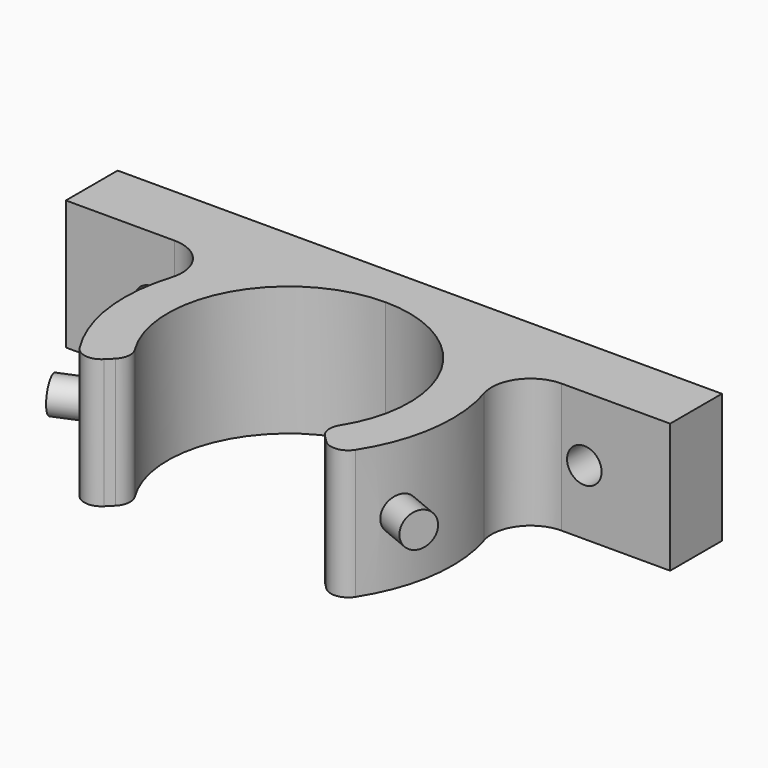
from build123d import *

# Parameters (mm, degrees)
F1_DEPTH  = 15
F2_R      = 2
F3_DEPTH  = 7.5
F4_ANGLE  = 90
F5_R      = 4.5
F6_R      = 2
F10_R     = 2
F11_DEPTH = 5


# Not quite as in the source:
# - a pattern or mirror of a feature is missing from the dataset's text; its kind, count and spacing are read off the source's solid


with BuildPart() as f1:
    # F0 (on Right) → F1 (new body)
    with BuildSketch(Plane.YZ):
        with BuildLine():
            ThreePointArc((-8.7152049129, 10.9565141959), (6.0822336037, 12.6097753505), (14, 0))
            ThreePointArc((14, 0), (6.0822336037, -12.6097753505), (-8.7152049129, -10.9565141959))
            Line((-8.7152049129, -10.9565141959), (-12.2675540951, -14.5088633781))
            ThreePointArc((-12.2675540951, -14.5088633781), (-0.4919673203, -18.993629673), (11.5, -15.1244834623))
            ThreePointArc((11.5, -15.1244834623), (17.0220445305, -8.4409715081), (19, 0))
            ThreePointArc((19, 0), (17.0220445305, 8.4409715081), (11.5, 15.1244834623))
            ThreePointArc((11.5, 15.1244834623), (-0.4919673203, 18.993629673), (-12.2675540951, 14.5088633781))
            Line((-12.2675540951, 14.5088633781), (-8.7152049129, 10.9565141959))
        make_face()
        with BuildLine():
            Line((11.5, 35), (11.5, 15.1244834623))
            ThreePointArc((11.5, 15.1244834623), (17.0220445305, 8.4409715081), (19, 0))
            Line((19, 0), (19, 35))
            Line((19, 35), (11.5, 35))
        make_face()
        with BuildLine():
            ThreePointArc((19, 0), (17.0220445305, -8.4409715081), (11.5, -15.1244834623))
            Line((11.5, -15.1244834623), (11.5, -35))
            Line((11.5, -35), (19, -35))
            Line((19, -35), (19, 0))
        make_face()
    extrude(amount=F1_DEPTH)

    # F2 (on face) → F3 (cut, through all)
    with BuildSketch(Plane.XZ.offset(-11.5)):
        with Locations((7.5, 25.0622417311)):
            Circle(F2_R)
        with Locations((7.5, -25.0622417311)):
            Circle(F2_R)
    extrude(amount=-F3_DEPTH, mode=Mode.SUBTRACT)


with BuildPart() as f1_1:
    # F4: moved
    add(f1.part.rotate(Axis((0, -7, 0), (0, -1, 0)), F4_ANGLE))

    # F5
    f5_edges = [f1_1.edges().sort_by_distance(p)[0] for p in [
        (-15.124483, 11.5, 7.5),
        (15.124483, 11.5, 7.5),
    ]]
    fillet(f5_edges, radius=F5_R)

    # F6
    f6_edges = [f1_1.edges().sort_by_distance(p)[0] for p in [
        (10.956514, -8.715205, 7.5),
        (-10.956514, -8.715205, 7.5),
        (-14.508863, -12.267554, 7.5),
        (14.508863, -12.267554, 7.5),
    ]]
    fillet(f6_edges, radius=F6_R)

    # F10 (on line) → F11 (join)
    with BuildSketch(Plane(origin=(16.2175144213, -6.7175144213, 0), x_dir=(-0.3826834324, -0.9238795325, 0), z_dir=(-0.9238795325, 0.3826834324, 0))):
        with Locations((-1.0217712261, 7.4956147)):
            Circle(F10_R)
    f11 = extrude(amount=-F11_DEPTH)

    # F11_copies: F11 across plane
    add(f11.mirror(Plane(origin=(0, 0, 0), x_dir=(0, 0, -1), z_dir=(-1, 0, 0))))


solid = f1_1.part
